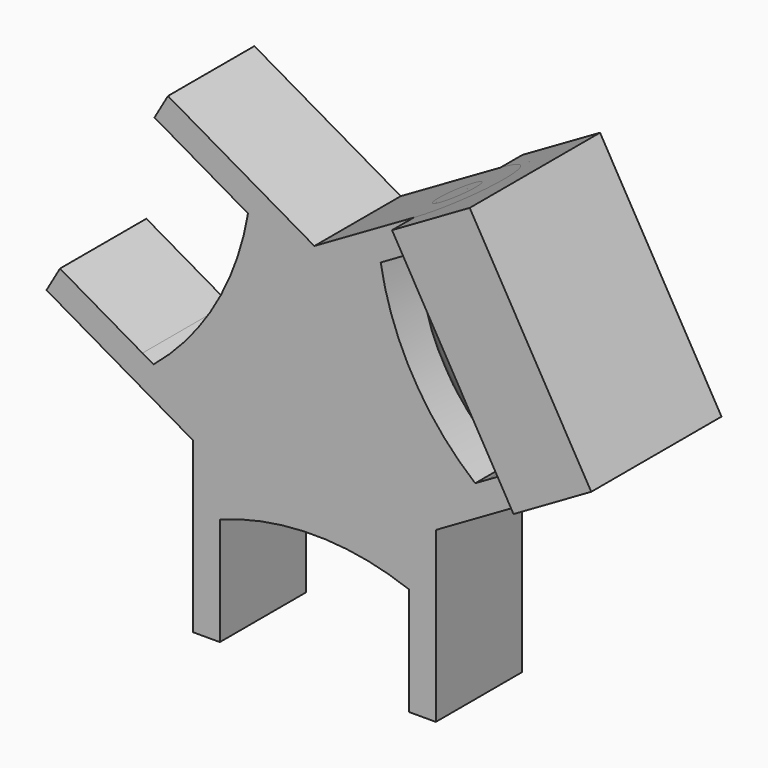
from build123d import *

# Parameters (mm, degrees)
F3_DEPTH = 6
F5_DEPTH = 27
F4_R     = 2.35


# Not quite as in the source:
# - a feature of the source that left no trace in its solid (it failed there, or was rolled back) is left out


with BuildPart() as f2:
    # F1 (on Front) → F2 (revolve)
    with BuildSketch(Plane.XZ):
        with BuildLine():
            Line((18.6924170284, -0.7549333807), (19.7635302092, -0.1365258974))
            Line((19.7635302092, -0.1365258974), (17.2635302092, 4.1936011215))
            Line((17.2635302092, 4.1936011215), (18.129555613, 4.6936011215))
            Line((18.129555613, 4.6936011215), (13.129555613, 13.3538551594))
            Line((13.129555613, 13.3538551594), (12.2635302092, 12.8538551594))
            Line((12.2635302092, 12.8538551594), (9.7635302092, 17.1839821783))
            Line((9.7635302092, 17.1839821783), (8.6924170284, 16.565574695))
            ThreePointArc((8.6924170284, 16.565574695), (12.2065523427, 7.0474562809), (18.6924170284, -0.7549333807))
        make_face()
    revolve(axis=Axis((19.0936572281, 0, 11.0237281405), (0.5, 0, -0.8660254038)))


with BuildPart() as f3:
    # F0 (on Front) → F3 (new body, symmetric)
    with BuildSketch(Plane.XZ):
        with BuildLine():
            Line((8.5998433468, 17.0894775242), (17.7628466203, 22.3797399308))
            Line((17.7628466203, 22.3797399308), (16.2628466203, 24.9778161421))
            Line((16.2628466203, 24.9778161421), (0, 15.5884572681))
            Line((0, 15.5884572681), (-16.2628466203, 24.9778161421))
            Line((-16.2628466203, 24.9778161421), (-17.7628466203, 22.3797399308))
            Line((-17.7628466203, 22.3797399308), (-8.5998433468, 17.0894775242))
            Line((-8.5998433468, 17.0894775242), (-7.3705417748, 16.3797399308))
            ThreePointArc((-7.3705417748, 16.3797399308), (-10.9772507707, 6.3377186874), (-17.8705417748, -1.8067935487))
            Line((-17.8705417748, -1.8067935487), (-19.0998433468, -1.0970559552))
            Line((-19.0998433468, -1.0970559552), (-28.2628466203, 4.1932064513))
            Line((-28.2628466203, 4.1932064513), (-29.7628466203, 1.5951302399))
            Line((-29.7628466203, 1.5951302399), (-13.5, -7.7942286341))
            Line((-13.5, -7.7942286341), (-13.5, -26.5729463821))
            Line((-13.5, -26.5729463821), (-10.5, -26.5729463821))
            Line((-10.5, -26.5729463821), (-10.5, -15.992421569))
            Line((-10.5, -15.992421569), (-10.5, -14.5729463821))
            ThreePointArc((-10.5, -14.5729463821), (0, -12.6754373748), (10.5, -14.5729463821))
            Line((10.5, -14.5729463821), (10.5, -15.992421569))
            Line((10.5, -15.992421569), (10.5, -26.5729463821))
            Line((10.5, -26.5729463821), (13.5, -26.5729463821))
            Line((13.5, -26.5729463821), (13.5, -7.7942286341))
            Line((13.5, -7.7942286341), (29.7628466203, 1.5951302399))
            Line((29.7628466203, 1.5951302399), (28.2628466203, 4.1932064513))
            Line((28.2628466203, 4.1932064513), (19.0998433468, -1.0970559552))
            Line((19.0998433468, -1.0970559552), (17.8705417748, -1.8067935487))
            ThreePointArc((17.8705417748, -1.8067935487), (10.9772507707, 6.3377186874), (7.3705417748, 16.3797399308))
            Line((7.3705417748, 16.3797399308), (8.5998433468, 17.0894775242))
        make_face()
    extrude(amount=F3_DEPTH, both=True)


with BuildPart() as f5:
    # F4 (on face) → F5 (new body)
    with BuildSketch(Plane(origin=(-6.75, 0, 11.6913429511), x_dir=(0.8660254038, 0, 0.5), z_dir=(-0.5, 0, 0.8660254038))):
        with BuildLine():
            ThreePointArc((20.5729463821, 6), (26.5729463821, 0), (20.5729463821, -6))
            Line((20.5729463821, -6), (20.5729463821, -9.0451398864))
            Line((20.5729463821, -9.0451398864), (30.5433310568, -9.0451398864))
            Line((30.5433310568, -9.0451398864), (30.5433310568, 9.0504763648))
            Line((30.5433310568, 9.0504763648), (20.5729463821, 9.0504763648))
            Line((20.5729463821, 9.0504763648), (20.5729463821, 6))
        make_face()
    extrude(amount=-F5_DEPTH)


with BuildPart() as f5b:
    # F4 (on face) → F5, piece 2 (new body)
    with BuildSketch(Plane(origin=(-6.75, 0, 11.6913429511), x_dir=(0.8660254038, 0, 0.5), z_dir=(-0.5, 0, 0.8660254038))):
        with Locations((20.5729463821, 0)):
            Circle(F4_R)
    extrude(amount=-F5_DEPTH)


solid = Compound([f2.part, f3.part, f5.part, f5b.part])
